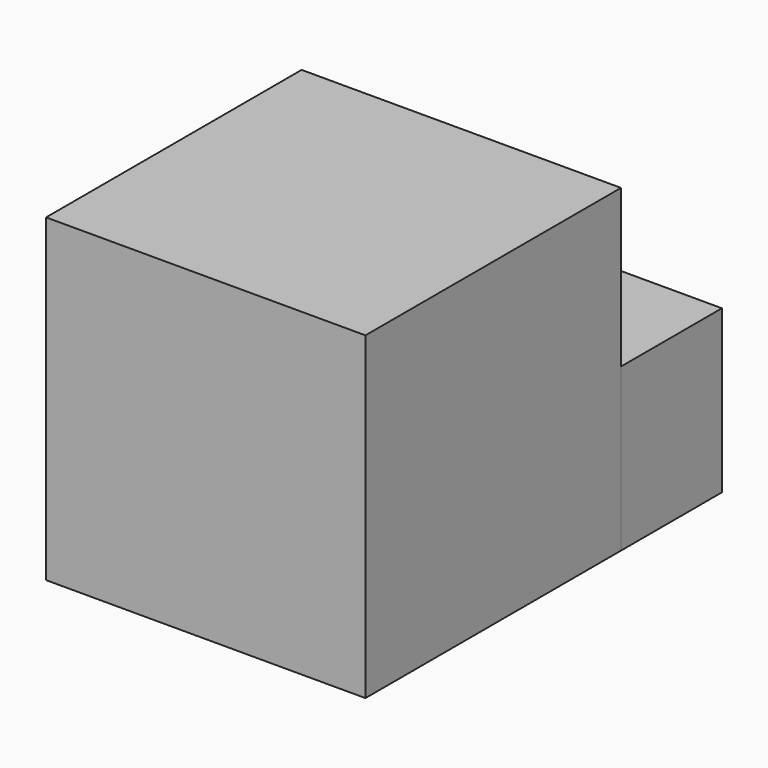
from build123d import *

# Parameters (mm, degrees)
F0_W     = 50.7939383388
F0_H     = 50.7939346135
F1_DEPTH = 50.8
F2_W     = 25.3969691694
F2_H     = 25.3969673067
F3_DEPTH = 25.4
F6_W     = 25.3969673067
F6_H     = 25.7788784802
F7_DEPTH = 20.066


# Not quite as in the source:
# - the program builds the solid bodies; features that only make, move or delete a surface that nothing else refers to are left out


with BuildPart() as f1:
    # F0 (on Front) → F1 (new body)
    with BuildSketch(Plane.XZ):
        with Locations((-25.3969691694, 25.3969673067)):
            Rectangle(F0_W, F0_H)
    extrude(amount=F1_DEPTH)

    # F2 (on Front) → F3 (join)
    with BuildSketch(Plane.XZ):
        with Locations((-38.0954537541, 12.6984836534)):
            Rectangle(F2_W, F2_H)
    extrude(amount=F3_DEPTH)


with BuildPart() as f7:
    # F6 (on Front) → F7 (new body)
    with BuildSketch(Plane.XZ):
        with Locations((-12.6984836534, 12.8894392401)):
            Rectangle(F6_W, F6_H)
    extrude(amount=-F7_DEPTH)


solid = Compound([f1.part, f7.part])
